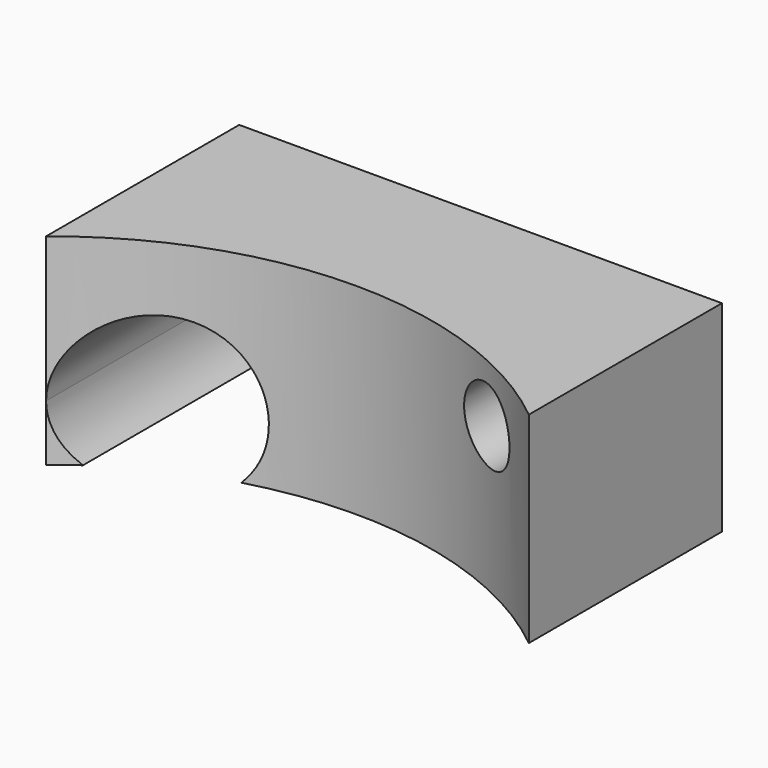
from build123d import *

# Parameters (mm, degrees)
F1_DEPTH = 25
F2_R     = 4.5
F3_REACH = 56.2498094968


with BuildPart() as f1:
    # F0 (on Top) → F1 (new body)
    with BuildSketch(Plane.XY):
        with BuildLine():
            Line((30, 15), (-30, 15))
            Line((-30, 15), (-30, -15))
            ThreePointArc((-30, -15), (0, -4.3244223472), (30, -15))
            Line((30, -15), (30, 15))
        make_face()
    extrude(amount=F1_DEPTH)

    f3_end = f1.faces().sort_by_distance((0, -4.3244223472, 12.5))[0]
    # F2 (on face) → F3 (cut, up to a face of the model that its end follows)
    with BuildSketch(Plane(origin=(0, 15, 0), x_dir=(-1, 0, 0), z_dir=(0, 1, 0))):
        with BuildLine():
            ThreePointArc((27.1414284285, 0), (29.2578151927, 3.2194103823), (30, 7))
            ThreePointArc((30, 7), (16.2194103823, 16.2578151927), (12.8585715715, 0))
            Line((12.8585715715, 0), (27.1414284285, 0))
        make_face()
        with Locations((-20, 18)):
            Circle(F2_R)
    f3_long = extrude(amount=-F3_REACH, mode=Mode.PRIVATE)
    add(split(f3_long, bisect_by=f3_end, keep=Keep.BOTTOM, mode=Mode.PRIVATE), mode=Mode.SUBTRACT)


solid = f1.part
